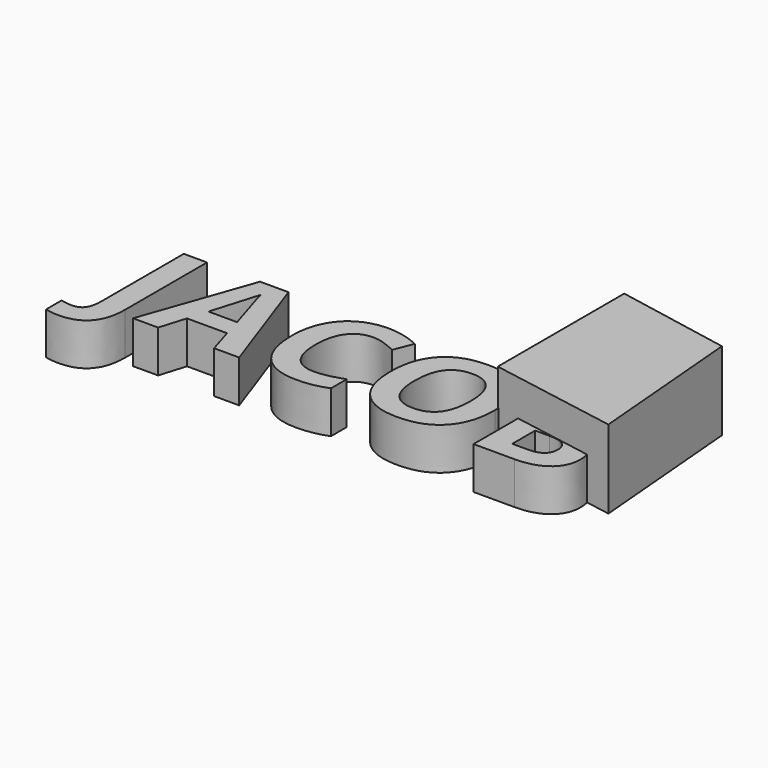
from build123d import *

# Parameters (mm, degrees)
F1_DEPTH     = 47.23351
F2_TEXT_SIZE = 92.6722125668
F3_DEPTH     = 25.4


# Not quite as in the source:
# - Text() gives the source's letters only with a copy of the font that has no kerning and outlines rounded to 1/6400 em; it was checked with that copy


with BuildPart() as f1:
    # F0 (on Top) → F1 (new body)
    with BuildSketch(Plane.XY):
        Polygon((130.5028349161, 64.0879422426), (61.1473061144, 77.2647038102), (61.1473061144, -17.9328396916), (138.6241316795, -31.5209515393), align=None)
    extrude(amount=F1_DEPTH)

    # F2 (on Top) → F3 (join)
    with BuildSketch(Plane.XY):
        with Locations((-160.3964269161, -53.9311282337)):
            Text('JACOB', F2_TEXT_SIZE, font='Open Sans', font_style=FontStyle.BOLD, text_align=(TextAlign.LEFT, TextAlign.BOTTOM))
    extrude(amount=F3_DEPTH)


solid = f1.part
